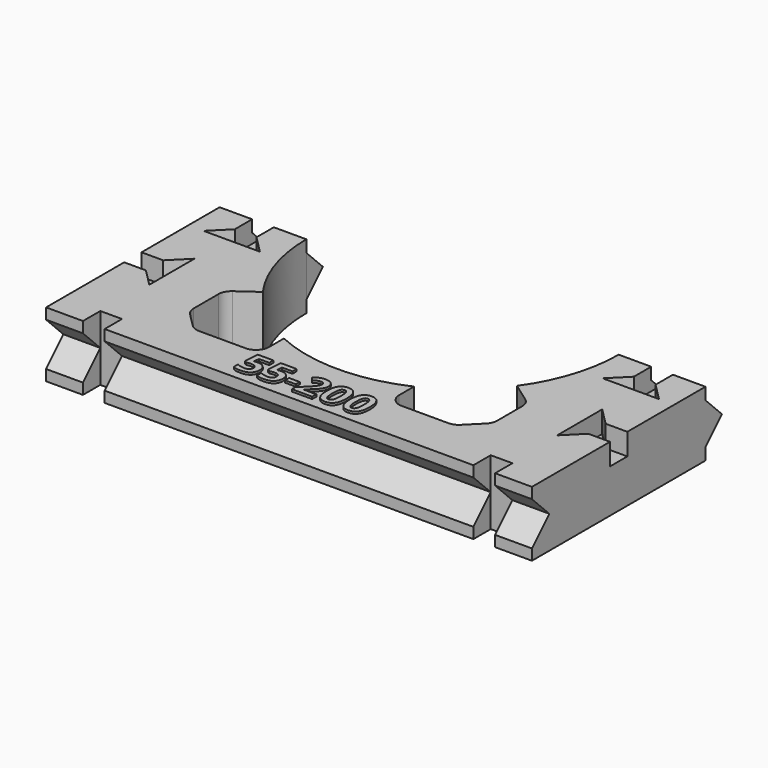
from build123d import *

# Parameters (mm, degrees)
F1_DEPTH      = 15
F2_SIZE       = 5
F3_R          = 3
F5_DEPTH      = 20
F7_DEPTH      = 20
F9_DEPTH      = 5
F11_DEPTH     = 112.001
F12_W         = 5
F12_H         = 5
F13_DEPTH     = 25
F15_DEPTH     = 5
F16_TEXT_SIZE = 9.3608307737
F17_DEPTH     = 0.5


# Not quite as in the source:
# - Text() gives the source's letters only with a copy of the font that has no kerning and outlines rounded to 1/6400 em; it was checked with that copy


with BuildPart() as f1:
    # F0 (on Top) → F1 (new body)
    with BuildSketch(Plane.XY):
        with BuildLine():
            Line((-56, 50), (-56, 0))
            Line((-56, 0), (56, 0))
            Line((56, 0), (56, 50))
            Line((56, 50), (36, 50))
            ThreePointArc((36, 50), (34.2826383078, 39.0136124837), (29.2944049634, 29.0754250261))
            Line((29.2944049634, 29.0754250261), (35, 25))
            Line((35, 25), (35, 10))
            Line((35, 10), (15, 10))
            Line((15, 10), (15, 17.2738636561))
            ThreePointArc((15, 17.2738636561), (0, 14), (-15, 17.2738636561))
            Line((-15, 17.2738636561), (-15, 10))
            Line((-15, 10), (-35, 10))
            Line((-35, 10), (-35, 25))
            Line((-35, 25), (-29.2944049634, 29.0754250261))
            ThreePointArc((-29.2944049634, 29.0754250261), (-34.2826383078, 39.0136124837), (-36, 50))
            Line((-36, 50), (-56, 50))
        make_face()
    extrude(amount=F1_DEPTH)

    # F2
    f2_edges = [f1.edges().sort_by_distance(p)[0] for p in [
        (-35, 10, 7.5),
        (35, 10, 7.5),
    ]]
    chamfer(f2_edges, length=F2_SIZE)

    # F3
    f3_edges = [f1.edges().sort_by_distance(p)[0] for p in [
        (-15, 10, 7.5),
        (-30, 10, 7.5),
        (-35, 15, 7.5),
        (-35, 25, 7.5),
        (15, 10, 7.5),
        (30, 10, 7.5),
        (35, 15, 7.5),
        (35, 25, 7.5),
    ]]
    fillet(f3_edges, radius=F3_R)

    # F4 (on face) → F5 (join)
    with BuildSketch(Plane(origin=(-56, 0, 0), x_dir=(0, -1, 0), z_dir=(-1, 0, 0))):
        Polygon((-54.75, 7.5), (-50, 2.75), (-50, 12.25), align=None)
    extrude(amount=-F5_DEPTH)

    # F6 (on face) → F7 (join)
    with BuildSketch(Plane.YZ.offset(56)):
        Polygon((50, 2.75), (54.75, 7.5), (50, 12.25), align=None)
    extrude(amount=-F7_DEPTH)

    # F8 (on face) → F9 (cut)
    with BuildSketch(Plane.XY.offset(15)):
        Polygon((-56, 27.5), (-56, 22.5), (-51, 22.5), (-47, 18.5), (-47, 31.5), (-51, 27.5), align=None)
        Polygon((47, 31.5), (47, 18.5), (51, 22.5), (56, 22.5), (56, 27.5), (51, 27.5), align=None)
    extrude(amount=-F9_DEPTH, mode=Mode.SUBTRACT)

    # F10 (on face) → F11 (cut, through all)
    with BuildSketch(Plane.YZ.offset(56)):
        Polygon((5, 7.5), (0, 12.5), (0, 2.5), align=None)
    extrude(amount=-F11_DEPTH, mode=Mode.SUBTRACT)

    # F12 (on face) → F13 (cut)
    with BuildSketch(Plane(origin=(0, 0, 0), x_dir=(1, 0, 0), z_dir=(0, 0, -1))):
        with Locations((45, -2.5)):
            Rectangle(F12_W, F12_H)
        with Locations((-45, -2.5)):
            Rectangle(F12_W, F12_H)
    extrude(amount=-F13_DEPTH, mode=Mode.SUBTRACT)

    # F14 (on face) → F15 (cut)
    with BuildSketch(Plane.XY.offset(15)):
        Polygon((-48.5, 45), (-52.5, 41), (-39.5, 41), (-43.5, 45), (-43.5, 50), (-43.5, 55.4240979254), (-48.5, 55.4240979254), (-48.5, 50), align=None)
        Polygon((48.5, 50), (48.5, 55.4240979254), (43.5, 55.4240979254), (43.5, 50), (43.5, 45), (39.5, 41), (52.5, 41), (48.5, 45), align=None)
    extrude(amount=-F15_DEPTH, mode=Mode.SUBTRACT)

    # F16 (on face) → F17 (join)
    with BuildSketch(Plane.XY.offset(15)):
        with Locations((-15, 2)):
            Text('55-200', F16_TEXT_SIZE, font='Open Sans', font_style=FontStyle.BOLD, text_align=(TextAlign.LEFT, TextAlign.BOTTOM))
    extrude(amount=F17_DEPTH)


solid = f1.part
